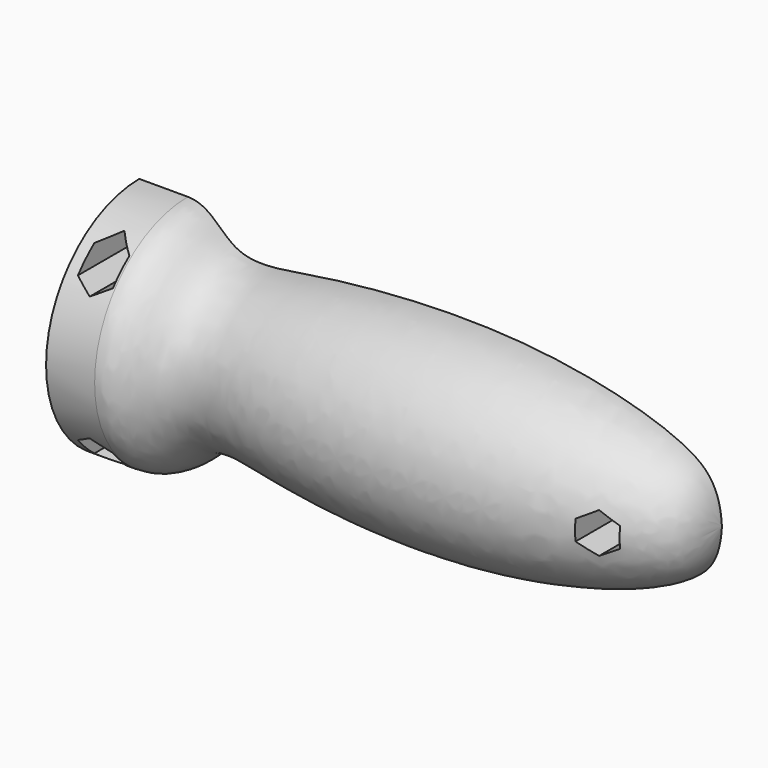
from build123d import *

# Parameters (mm, degrees)
F1_ANGLE = 180
F3_D     = 4.4
F6_R     = 2.2
F7_DEPTH = 19


with BuildPart() as f1:
    # F0 (on Front) → F1 (revolve)
    with BuildSketch(Plane.XZ):
        with BuildLine():
            Line((0, 24), (0, 13))
            Line((0, 13), (53, 13))
            Line((53, 13), (53, 17))
            Line((53, 17), (64, 17))
            Line((64, 17), (64, 13))
            Line((64, 13), (100, 13))
            Line((100, 13), (100, 0))
            Line((100, 0), (120, 0))
            add(Edge.make_bspline(
                [(10, 24), (14.5846361259, 24), (19.1911767131, 14.7073521681), (38.5291539725, 19.2623560501), (77.4336550451, 22.1476524592), (112.1829708833, 14.2248736546), (119.6026350157, 7.3835916313), (120, 0)],
                knots=[0, 0, 0, 0, 0.1438984957, 0.3179448336, 0.5884486431, 0.835948418, 1, 1, 1, 1], degree=3))
            Line((10, 24), (0, 24))
        make_face()
    revolve(axis=Axis((50, 0, 0), (1, 0, 0)), revolution_arc=F1_ANGLE)

    # F3 (through all)
    with Locations(Plane(origin=(0, 0, 0), x_dir=(1, 0, 0), z_dir=(0, 1, 0))):
        with Locations((6, -17), (6, 17), (106, 0)):
            Hole(F3_D / 2)

    # F6 (on plane+point) → F7 (cut)
    with BuildSketch(Plane.XZ.offset(24)):
        Polygon((9.6, 14.9215390309), (9.6, 19.0784609691), (6, 21.1569219382), (2.4, 19.0784609691), (2.4, 14.9215390309), (6, 12.8430780618), align=None)
        with Locations((6, 17)):
            Circle(F6_R, mode=Mode.SUBTRACT)
        Polygon((9.6, -19.0784609691), (9.6, -14.9215390309), (6, -12.8430780618), (2.4, -14.9215390309), (2.4, -19.0784609691), (6, -21.1569219382), align=None)
        with Locations((6, -17)):
            Circle(F6_R, mode=Mode.SUBTRACT)
        Polygon((109.6, -2.0784609691), (109.6, 2.0784609691), (106, 4.1569219382), (102.4, 2.0784609691), (102.4, -2.0784609691), (106, -4.1569219382), align=None)
        with Locations((106, 0)):
            Circle(F6_R, mode=Mode.SUBTRACT)
    extrude(amount=-F7_DEPTH, mode=Mode.SUBTRACT)


solid = f1.part
